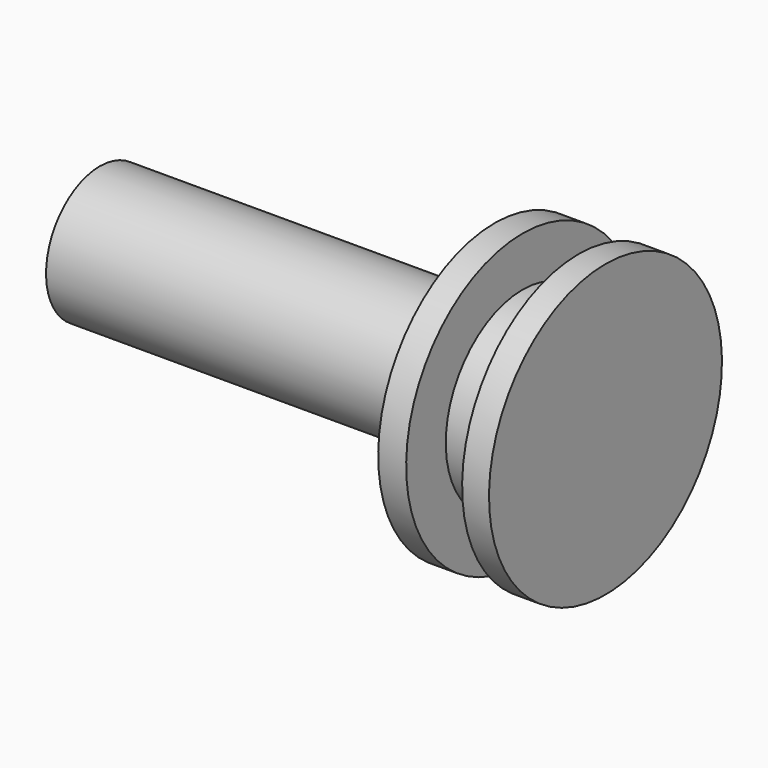
from build123d import *


# Not quite as in the source:
# - a fillet or chamfer that OpenCascade refuses, or shapes differently, is made with other operations: its cross-section is extruded or revolved along the edge and cut away or added


with BuildPart() as f1:
    # F0 (on Front) → F1 (revolve)
    with BuildSketch(Plane.XZ):
        Polygon((-35.814, 0), (0, 0), (0, 10.3124), (-1.905, 10.3124), (-1.905, 6.8072), (-5.8674, 6.8072), (-5.8674, 10.3124), (-7.8486, 10.3124), (-7.8486, 3.9243), (-9.7536, 3.9243), (-9.7536, 4.7625), (-35.814, 4.7625), align=None)
    revolve(axis=Axis((-27.8073139489, 0, 0), (-1, 0, 0)))

    # F2: fillet of radius 0.9398 on 2 edges, made by hand

    # F2_s1 → F2_t2 (revolve)
    with BuildSketch(Plane.XZ):
        with BuildLine():
            ThreePointArc((-7.8486, 4.8641), (-8.123861047, 4.199561047), (-8.7884, 3.9243))
            Line((-8.7884, 3.9243), (-7.8486, 3.9243))
            Line((-7.8486, 3.9243), (-7.8486, 4.8641))
        make_face()
    revolve(axis=Axis((-7.8486, 0, 0), (-1, 0, 0)))

    # F2_s3 → F2_t4 (revolve)
    with BuildSketch(Plane.XZ):
        with BuildLine():
            ThreePointArc((-8.8193080328, 3.9243), (-9.4468988071, 4.1645616808), (-9.7536, 4.7625))
            Line((-9.7536, 4.7625), (-9.7536, 3.9243))
            Line((-9.7536, 3.9243), (-8.8193080328, 3.9243))
        make_face()
    revolve(axis=Axis((-9.7536, 0, 0), (-1, 0, 0)))


solid = f1.part
